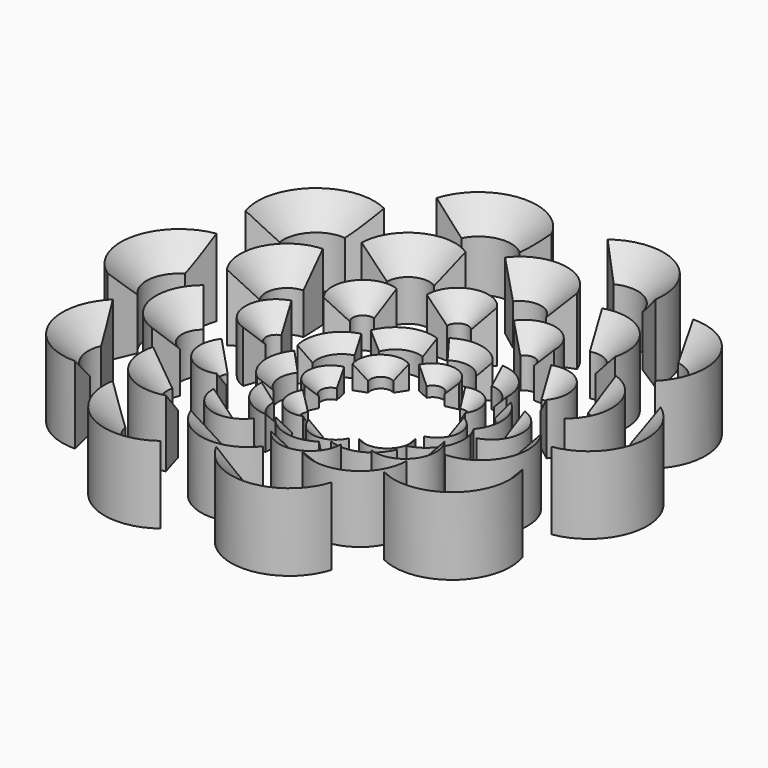
from build123d import *

# Parameters (mm, degrees)
F2_DEPTH       = 15
F3_DEPTH       = 13
F4_DEPTH       = 11
F5_DEPTH       = 9
F6_DEPTH       = 7
F7_T2_ANGLE    = 336.4519839088
F7_2_T2_ANGLE  = 359.64
F7_3_T2_ANGLE  = 336.4519839088
F7_4_T2_ANGLE  = 359.64
F7_5_T2_ANGLE  = 336.4519839088
F7_6_T2_ANGLE  = 336.4519839088
F7_7_T2_ANGLE  = 359.64
F7_8_T2_ANGLE  = 359.64
F7_9_T2_ANGLE  = 359.64
F7_10_T2_ANGLE = 359.64
F7_11_T2_ANGLE = 359.64
F7_12_T2_ANGLE = 359.64
F7_13_T2_ANGLE = 359.64
F7_14_T2_ANGLE = 336.4519839088
F7_15_T2_ANGLE = 336.4519839088
F7_16_T2_ANGLE = 359.64
F7_17_T2_ANGLE = 336.4519839088
F7_18_T2_ANGLE = 336.4519839088
F7_19_T2_ANGLE = 359.64
F7_20_T2_ANGLE = 359.64
F7_21_T2_ANGLE = 359.64
F7_22_T2_ANGLE = 359.64
F7_23_T2_ANGLE = 336.4519839088
F7_24_T2_ANGLE = 359.64
F7_25_T2_ANGLE = 359.64
F7_26_T2_ANGLE = 336.4519839088
F7_27_T2_ANGLE = 359.64
F7_28_T2_ANGLE = 359.64
F7_29_T2_ANGLE = 359.64
F7_30_T2_ANGLE = 359.64
F7_31_T2_ANGLE = 359.64
F7_32_T2_ANGLE = 359.64
F7_33_T2_ANGLE = 359.64
F7_34_T2_ANGLE = 359.64
F7_35_T2_ANGLE = 359.64
F7_36_T2_ANGLE = 359.64
F7_37_T2_ANGLE = 359.64
F7_38_T2_ANGLE = 359.64
F7_39_T2_ANGLE = 359.64
F7_40_T2_ANGLE = 359.64
F7_41_T2_ANGLE = 359.64
F7_42_T2_ANGLE = 359.64
F7_43_T2_ANGLE = 359.64
F7_44_T2_ANGLE = 359.64
F7_45_T2_ANGLE = 359.64
F7_46_T2_ANGLE = 359.64
F7_47_T2_ANGLE = 359.64
F7_48_T2_ANGLE = 359.64


# Not quite as in the source:
# - a fillet or chamfer that OpenCascade refuses, or shapes differently, is made with other operations: its cross-section is extruded or revolved along the edge and cut away or added


with BuildPart() as f2:
    # F1 (on offset) → F2 (new body)
    with BuildSketch(Plane.XY.offset(30)):
        with BuildLine():
            ThreePointArc((17.7590144577, -41.0240965166), (13.3006914412, -44.3521341763), (7.933868463, -42.8859520918))
            Line((7.933868463, -42.8859520918), (1.9961113601, -43.2368292953))
            ThreePointArc((1.9961113601, -43.2368292953), (13.0634500325, -49.4237184718), (22.9515977997, -41.487213151))
            Line((22.9515977997, -41.487213151), (17.7590144577, -41.0240965166))
        make_face()
    extrude(amount=F2_DEPTH)

    # F7#6: chamfer of 5 on 1 edges, made by hand

    # F7_6_s1 → F7_6_t2 (revolve, cut)
    with BuildSketch(Plane(origin=(12.8099025435, -0.2333815755, 0), x_dir=(0, 0, 1), z_dir=(-0.9998340782, 0.0182158179, 0))):
        Polygon((40, -31.5493184866), (45, -26.5493184866), (45, -31.5493184866), align=None)
    revolve(axis=Axis((12.1196571692, -38.1197312438, 45), (0, 0, -1)), revolution_arc=F7_6_T2_ANGLE, mode=Mode.SUBTRACT)


with BuildPart() as f2b:
    # F1 (on offset) → F2, piece 2 (new body)
    with BuildSketch(Plane.XY.offset(30)):
        with BuildLine():
            ThreePointArc((-9.7460144214, -43.6276780543), (-15.3090449637, -43.6995805599), (-18.7890957524, -39.3588749384))
            Line((-18.7890957524, -39.3588749384), (-23.7990826027, -36.1526145022))
            ThreePointArc((-23.7990826027, -36.1526145022), (-18.4819797497, -47.663131442), (-5.8173393808, -47.0544711917))
            Line((-5.8173393808, -47.0544711917), (-9.7460144214, -43.6276780543))
        make_face()
    extrude(amount=F2_DEPTH)

    # F7#5: chamfer of 5 on 1 edges, made by hand

    # F7_5_s1 → F7_5_t2 (revolve, cut)
    with BuildSketch(Plane(origin=(10.2262506057, -7.7182814591, 0), x_dir=(0, 0, 1), z_dir=(-0.7981757717, 0.6024246322, 0))):
        Polygon((40, -31.5493184866), (45, -26.5493184866), (45, -31.5493184866), align=None)
    revolve(axis=Axis((-12.6012072306, -37.9632661442, 45), (0, 0, -1)), revolution_arc=F7_5_T2_ANGLE, mode=Mode.SUBTRACT)


with BuildPart() as f2c:
    # F1 (on offset) → F2, piece 3 (new body)
    with BuildSketch(Plane.XY.offset(30)):
        with BuildLine():
            ThreePointArc((-33.5283970464, -29.5669694255), (-38.0712465277, -26.3552724637), (-38.3352640082, -20.7980453175))
            Line((-38.3352640082, -20.7980453175), (-40.5038359123, -15.2593297514))
            ThreePointArc((-40.5038359123, -15.2593297514), (-42.9679214469, -27.6968482117), (-32.364250642, -34.6485205598))
            Line((-32.364250642, -34.6485205598), (-33.5283970464, -29.5669694255))
        make_face()
    extrude(amount=F2_DEPTH)

    # F7#3: chamfer of 5 on 1 edges, made by hand

    # F7_3_s1 → F7_3_t2 (revolve, cut)
    with BuildSketch(Plane(origin=(3.7365185141, -12.2550601601, 0), x_dir=(0, 0, 1), z_dir=(-0.2916414494, 0.9565277126, 0))):
        Polygon((40, -31.5493184866), (45, -26.5493184866), (45, -31.5493184866), align=None)
    revolve(axis=Axis((-32.5088387676, -23.3061237014, 45), (0, 0, -1)), revolution_arc=F7_3_T2_ANGLE, mode=Mode.SUBTRACT)


with BuildPart() as f2d:
    # F1 (on offset) → F2, piece 4 (new body)
    with BuildSketch(Plane.XY.offset(30)):
        with BuildLine():
            ThreePointArc((-44.504071588, -4.2126834205), (-46.2915259123, 1.0558539309), (-43.2386643806, 5.7069307151))
            Line((-43.2386643806, 5.7069307151), (-41.7375005782, 11.4625003189))
            ThreePointArc((-41.7375005782, 11.4625003189), (-51.0415775773, 2.8486896542), (-46.5491181784, -9.0080127339))
            Line((-46.5491181784, -9.0080127339), (-44.504071588, -4.2126834205))
        make_face()
    extrude(amount=F2_DEPTH)

    # F7: chamfer of 5 on 1 edges, made by hand

    # F7_s1 → F7_t2 (revolve, cut)
    with BuildSketch(Plane(origin=(-4.1804366504, -12.1108224141, 0), x_dir=(0, 0, 1), z_dir=(0.3262899941, 0.945269718, 0))):
        Polygon((40, -31.5493184866), (45, -26.5493184866), (45, -31.5493184866), align=None)
    revolve(axis=Axis((-39.9991988301, 0.2531658493, 45), (0, 0, -1)), revolution_arc=F7_T2_ANGLE, mode=Mode.SUBTRACT)


with BuildPart() as f2e:
    # F1 (on offset) → F2, piece 5 (new body)
    with BuildSketch(Plane.XY.offset(30)):
        with BuildLine():
            ThreePointArc((-38.4807034207, 22.7507044673), (-36.8300157894, 28.063680011), (-31.6263645878, 30.032053186))
            Line((-31.6263645878, 30.032053186), (-27.0288586286, 33.8060448634))
            ThreePointArc((-27.0288586286, 33.8060448634), (-39.6190859126, 32.3061248957), (-42.9538047169, 20.0732497852))
            Line((-42.9538047169, 20.0732497852), (-38.4807034207, 22.7507044673))
        make_face()
    extrude(amount=F2_DEPTH)

    # F7#14: chamfer of 5 on 1 edges, made by hand

    # F7_14_s1 → F7_14_t2 (revolve, cut)
    with BuildSketch(Plane(origin=(-10.5006071022, -7.3406621376, 0), x_dir=(0, 0, 1), z_dir=(0.81958975, 0.5729508196, 0))):
        Polygon((40, -31.5493184866), (45, -26.5493184866), (45, -31.5493184866), align=None)
    revolve(axis=Axis((-32.2112244624, 23.7157546503, 45), (0, 0, -1)), revolution_arc=F7_14_T2_ANGLE, mode=Mode.SUBTRACT)


with BuildPart() as f2f:
    # F1 (on offset) → F2, piece 6 (new body)
    with BuildSketch(Plane.XY.offset(30)):
        with BuildLine():
            ThreePointArc((-17.7590144577, 41.0240965166), (-13.3006914412, 44.3521341763), (-7.933868463, 42.8859520918))
            Line((-7.933868463, 42.8859520918), (-1.9961113601, 43.2368292953))
            ThreePointArc((-1.9961113601, 43.2368292953), (-13.0634500325, 49.4237184718), (-22.9515977997, 41.487213151))
            Line((-22.9515977997, 41.487213151), (-17.7590144577, 41.0240965166))
        make_face()
    extrude(amount=F2_DEPTH)

    # F7#15: chamfer of 5 on 1 edges, made by hand

    # F7_15_s1 → F7_15_t2 (revolve, cut)
    with BuildSketch(Plane(origin=(-12.8099025435, 0.2333815755, 0), x_dir=(0, 0, 1), z_dir=(0.9998340782, -0.0182158179, 0))):
        Polygon((40, -31.5493184866), (45, -26.5493184866), (45, -31.5493184866), align=None)
    revolve(axis=Axis((-12.1196571692, 38.1197312438, 45), (0, 0, -1)), revolution_arc=F7_15_T2_ANGLE, mode=Mode.SUBTRACT)


with BuildPart() as f2g:
    # F1 (on offset) → F2, piece 7 (new body)
    with BuildSketch(Plane.XY.offset(30)):
        with BuildLine():
            ThreePointArc((9.7460144214, 43.6276780543), (15.3090449637, 43.6995805599), (18.7890957524, 39.3588749384))
            Line((18.7890957524, 39.3588749384), (23.7990826027, 36.1526145022))
            ThreePointArc((23.7990826027, 36.1526145022), (18.4819797497, 47.663131442), (5.8173393808, 47.0544711917))
            Line((5.8173393808, 47.0544711917), (9.7460144214, 43.6276780543))
        make_face()
    extrude(amount=F2_DEPTH)

    # F7#17: chamfer of 5 on 1 edges, made by hand

    # F7_17_s1 → F7_17_t2 (revolve, cut)
    with BuildSketch(Plane(origin=(-10.2262506057, 7.7182814591, 0), x_dir=(0, 0, 1), z_dir=(0.7981757717, -0.6024246322, 0))):
        Polygon((40, -31.5493184866), (45, -26.5493184866), (45, -31.5493184866), align=None)
    revolve(axis=Axis((12.6012072306, 37.9632661442, 45), (0, 0, -1)), revolution_arc=F7_17_T2_ANGLE, mode=Mode.SUBTRACT)


with BuildPart() as f2h:
    # F1 (on offset) → F2, piece 8 (new body)
    with BuildSketch(Plane.XY.offset(30)):
        with BuildLine():
            ThreePointArc((33.5283970464, 29.5669694255), (38.0712465277, 26.3552724637), (38.3352640082, 20.7980453175))
            Line((38.3352640082, 20.7980453175), (40.5038359123, 15.2593297514))
            ThreePointArc((40.5038359123, 15.2593297514), (42.9679214469, 27.6968482117), (32.364250642, 34.6485205598))
            Line((32.364250642, 34.6485205598), (33.5283970464, 29.5669694255))
        make_face()
    extrude(amount=F2_DEPTH)

    # F7#18: chamfer of 5 on 1 edges, made by hand

    # F7_18_s1 → F7_18_t2 (revolve, cut)
    with BuildSketch(Plane(origin=(-3.7365185141, 12.2550601601, 0), x_dir=(0, 0, 1), z_dir=(0.2916414494, -0.9565277126, 0))):
        Polygon((40, -31.5493184866), (45, -26.5493184866), (45, -31.5493184866), align=None)
    revolve(axis=Axis((32.5088387676, 23.3061237014, 45), (0, 0, -1)), revolution_arc=F7_18_T2_ANGLE, mode=Mode.SUBTRACT)


with BuildPart() as f2i:
    # F1 (on offset) → F2, piece 9 (new body)
    with BuildSketch(Plane.XY.offset(30)):
        with BuildLine():
            ThreePointArc((44.504071588, 4.2126834205), (46.2915259123, -1.0558539309), (43.2386643806, -5.7069307151))
            Line((43.2386643806, -5.7069307151), (41.7375005782, -11.4625003189))
            ThreePointArc((41.7375005782, -11.4625003189), (51.0415775773, -2.8486896542), (46.5491181784, 9.0080127339))
            Line((46.5491181784, 9.0080127339), (44.504071588, 4.2126834205))
        make_face()
    extrude(amount=F2_DEPTH)

    # F7#23: chamfer of 5 on 1 edges, made by hand

    # F7_23_s1 → F7_23_t2 (revolve, cut)
    with BuildSketch(Plane(origin=(4.1804366504, 12.1108224141, 0), x_dir=(0, 0, 1), z_dir=(-0.3262899941, -0.945269718, 0))):
        Polygon((40, -31.5493184866), (45, -26.5493184866), (45, -31.5493184866), align=None)
    revolve(axis=Axis((39.9991988301, -0.2531658493, 45), (0, 0, -1)), revolution_arc=F7_23_T2_ANGLE, mode=Mode.SUBTRACT)


with BuildPart() as f2j:
    # F1 (on offset) → F2, piece 10 (new body)
    with BuildSketch(Plane.XY.offset(30)):
        with BuildLine():
            ThreePointArc((38.4807034207, -22.7507044673), (36.8300157894, -28.063680011), (31.6263645878, -30.032053186))
            Line((31.6263645878, -30.032053186), (27.0288586286, -33.8060448634))
            ThreePointArc((27.0288586286, -33.8060448634), (39.6190859126, -32.3061248957), (42.9538047169, -20.0732497852))
            Line((42.9538047169, -20.0732497852), (38.4807034207, -22.7507044673))
        make_face()
    extrude(amount=F2_DEPTH)

    # F7#26: chamfer of 5 on 1 edges, made by hand

    # F7_26_s1 → F7_26_t2 (revolve, cut)
    with BuildSketch(Plane(origin=(10.5006071022, 7.3406621376, 0), x_dir=(0, 0, 1), z_dir=(-0.81958975, -0.5729508196, 0))):
        Polygon((40, -31.5493184866), (45, -26.5493184866), (45, -31.5493184866), align=None)
    revolve(axis=Axis((32.2112244624, -23.7157546503, 45), (0, 0, -1)), revolution_arc=F7_26_T2_ANGLE, mode=Mode.SUBTRACT)


with BuildPart() as f3:
    # F1 (on offset) → F3 (new body)
    with BuildSketch(Plane.XY.offset(30)):
        with BuildLine():
            Line((-6.1605418312, -31.6157678777), (-10.8426337183, -33.3701952944))
            ThreePointArc((-10.8426337183, -33.3701952944), (-3.5878071118, -39.2281581741), (5.0480977361, -35.7111444343))
            Line((5.0480977361, -35.7111444343), (1.0708378352, -32.6810613199))
            ThreePointArc((1.0708378352, -32.6810613199), (-2.8590949623, -34.2815453327), (-6.1605418312, -31.6157678777))
        make_face()
    extrude(amount=F3_DEPTH)

    # F7#7: chamfer of 5 on 1 edges, made by hand

    # F7_7_s1 → F7_7_t2 (revolve, cut)
    with BuildSketch(Plane(origin=(2.2372338796, -0.3367633156, 0), x_dir=(0, 0, 1), z_dir=(-0.9888598236, 0.1488497541, 0))):
        Polygon((38, -25.9742910378), (43, -20.9742910378), (43, -25.9742910378), align=None)
    revolve(axis=Axis((-2.2505512341, -30.1506546616, 43), (0, 0, -1)), revolution_arc=F7_7_T2_ANGLE, mode=Mode.SUBTRACT)


with BuildPart() as f3b:
    # F1 (on offset) → F3, piece 2 (new body)
    with BuildSketch(Plane.XY.offset(30)):
        with BuildLine():
            Line((-23.5672651344, -21.9566178688), (-28.3863836021, -20.6239149032))
            ThreePointArc((-28.3863836021, -20.6239149032), (-25.9603297754, -29.6273865125), (-16.9064871832, -31.8581201373))
            Line((-16.9064871832, -31.8581201373), (-18.3431198662, -27.0689566891))
            ThreePointArc((-18.3431198662, -27.0689566891), (-22.4632431853, -26.0538189138), (-23.5672651344, -21.9566178688))
        make_face()
    extrude(amount=F3_DEPTH)

    # F7#4: chamfer of 5 on 1 edges, made by hand

    # F7_4_s1 → F7_4_t2 (revolve, cut)
    with BuildSketch(Plane(origin=(1.6120157185, -1.5874603257, 0), x_dir=(0, 0, 1), z_dir=(-0.7125127121, 0.7016592016, 0))):
        Polygon((38, -25.9742910378), (43, -20.9742910378), (43, -25.9742910378), align=None)
    revolve(axis=Axis((-19.5428443521, -23.0695511878, 43), (0, 0, -1)), revolution_arc=F7_4_T2_ANGLE, mode=Mode.SUBTRACT)


with BuildPart() as f3c:
    # F1 (on offset) → F3, piece 3 (new body)
    with BuildSketch(Plane.XY.offset(30)):
        with BuildLine():
            Line((-31.9720941781, -3.910786112), (-35.0874997675, 0))
            ThreePointArc((-35.0874997675, 0), (-38.4168888238, -8.7099602009), (-32.4033686289, -15.8363767656))
            Line((-32.4033686289, -15.8363767656), (-30.7506292384, -11.1174306431))
            ThreePointArc((-30.7506292384, -11.1174306431), (-33.4871960092, -7.8744192066), (-31.9720941781, -3.910786112))
        make_face()
    extrude(amount=F3_DEPTH)

    # F7#2: chamfer of 5 on 1 edges, made by hand

    # F7_2_s1 → F7_2_t2 (revolve, cut)
    with BuildSketch(Plane(origin=(0.3710623434, -2.2318014472, 0), x_dir=(0, 0, 1), z_dir=(-0.164009962, 0.9864586826, 0))):
        Polygon((38, -25.9742910378), (43, -20.9742910378), (43, -25.9742910378), align=None)
    revolve(axis=Axis((-29.3704351645, -7.1766632655, 43), (0, 0, -1)), revolution_arc=F7_2_T2_ANGLE, mode=Mode.SUBTRACT)


with BuildPart() as f3d:
    # F1 (on offset) → F3, piece 4 (new body)
    with BuildSketch(Plane.XY.offset(30)):
        with BuildLine():
            Line((-28.1646699373, 15.6288330169), (-28.3863836021, 20.6239149032))
            ThreePointArc((-28.3863836021, 20.6239149032), (-36.1995020836, 15.5343748668), (-35.5232646083, 6.2343242719))
            Line((-35.5232646083, 6.2343242719), (-31.412443417, 9.080576041))
            ThreePointArc((-31.412443417, 9.080576041), (-31.7201781454, 13.3127409958), (-28.1646699373, 15.6288330169))
        make_face()
    extrude(amount=F3_DEPTH)

    # F7#12: chamfer of 5 on 1 edges, made by hand

    # F7_12_s1 → F7_12_t2 (revolve, cut)
    with BuildSketch(Plane(origin=(-1.0116242349, -2.023670272, 0), x_dir=(0, 0, 1), z_dir=(0.4471390191, 0.8944644753, 0))):
        Polygon((38, -25.9742910378), (43, -20.9742910378), (43, -25.9742910378), align=None)
    revolve(axis=Axis((-27.9795180084, 11.4574660984, 43), (0, 0, -1)), revolution_arc=F7_12_T2_ANGLE, mode=Mode.SUBTRACT)


with BuildPart() as f3e:
    # F1 (on offset) → F3, piece 5 (new body)
    with BuildSketch(Plane.XY.offset(30)):
        with BuildLine():
            Line((-13.5992990624, 29.1987691378), (-10.8426337183, 33.3701952944))
            ThreePointArc((-10.8426337183, 33.3701952944), (-20.1551359233, 33.8451067293), (-25.0744808987, 25.9237253345))
            Line((-25.0744808987, 25.9237253345), (-20.07577188, 25.8101113149))
            ThreePointArc((-20.07577188, 25.8101113149), (-17.8371303593, 29.4148866213), (-13.5992990624, 29.1987691378))
        make_face()
    extrude(amount=F3_DEPTH)

    # F7#13: chamfer of 5 on 1 edges, made by hand

    # F7_13_s1 → F7_13_t2 (revolve, cut)
    with BuildSketch(Plane(origin=(-2.0079047394, -1.0425658349, 0), x_dir=(0, 0, 1), z_dir=(0.8874960926, 0.4608152402, 0))):
        Polygon((38, -25.9742910378), (43, -20.9742910378), (43, -25.9742910378), align=None)
    revolve(axis=Axis((-15.901375962, 25.7152328377, 43), (0, 0, -1)), revolution_arc=F7_13_T2_ANGLE, mode=Mode.SUBTRACT)


with BuildPart() as f3f:
    # F1 (on offset) → F3, piece 6 (new body)
    with BuildSketch(Plane.XY.offset(30)):
        with BuildLine():
            Line((6.1605418312, 31.6157678777), (10.8426337183, 33.3701952944))
            ThreePointArc((10.8426337183, 33.3701952944), (3.5878071118, 39.2281581741), (-5.0480977361, 35.7111444343))
            Line((-5.0480977361, 35.7111444343), (-1.0708378352, 32.6810613199))
            ThreePointArc((-1.0708378352, 32.6810613199), (2.8590949623, 34.2815453327), (6.1605418312, 31.6157678777))
        make_face()
    extrude(amount=F3_DEPTH)

    # F7#16: chamfer of 5 on 1 edges, made by hand

    # F7_16_s1 → F7_16_t2 (revolve, cut)
    with BuildSketch(Plane(origin=(-2.2372338796, 0.3367633156, 0), x_dir=(0, 0, 1), z_dir=(0.9888598236, -0.1488497541, 0))):
        Polygon((38, -25.9742910378), (43, -20.9742910378), (43, -25.9742910378), align=None)
    revolve(axis=Axis((2.2505512341, 30.1506546616, 43), (0, 0, -1)), revolution_arc=F7_16_T2_ANGLE, mode=Mode.SUBTRACT)


with BuildPart() as f3g:
    # F1 (on offset) → F3, piece 7 (new body)
    with BuildSketch(Plane.XY.offset(30)):
        with BuildLine():
            Line((23.5672651344, 21.9566178688), (28.3863836021, 20.6239149032))
            ThreePointArc((28.3863836021, 20.6239149032), (25.9603297754, 29.6273865125), (16.9064871832, 31.8581201373))
            Line((16.9064871832, 31.8581201373), (18.3431198662, 27.0689566891))
            ThreePointArc((18.3431198662, 27.0689566891), (22.4632431853, 26.0538189138), (23.5672651344, 21.9566178688))
        make_face()
    extrude(amount=F3_DEPTH)

    # F7#19: chamfer of 5 on 1 edges, made by hand

    # F7_19_s1 → F7_19_t2 (revolve, cut)
    with BuildSketch(Plane(origin=(-1.6120157185, 1.5874603257, 0), x_dir=(0, 0, 1), z_dir=(0.7125127121, -0.7016592016, 0))):
        Polygon((38, -25.9742910378), (43, -20.9742910378), (43, -25.9742910378), align=None)
    revolve(axis=Axis((19.5428443521, 23.0695511878, 43), (0, 0, -1)), revolution_arc=F7_19_T2_ANGLE, mode=Mode.SUBTRACT)


with BuildPart() as f3h:
    # F1 (on offset) → F3, piece 8 (new body)
    with BuildSketch(Plane.XY.offset(30)):
        with BuildLine():
            Line((31.9720941781, 3.910786112), (35.0874997675, 0))
            ThreePointArc((35.0874997675, 0), (38.4168888238, 8.7099602009), (32.4033686289, 15.8363767656))
            Line((32.4033686289, 15.8363767656), (30.7506292384, 11.1174306431))
            ThreePointArc((30.7506292384, 11.1174306431), (33.4871960092, 7.8744192066), (31.9720941781, 3.910786112))
        make_face()
    extrude(amount=F3_DEPTH)

    # F7#22: chamfer of 5 on 1 edges, made by hand

    # F7_22_s1 → F7_22_t2 (revolve, cut)
    with BuildSketch(Plane(origin=(-0.3710623434, 2.2318014472, 0), x_dir=(0, 0, 1), z_dir=(0.164009962, -0.9864586826, 0))):
        Polygon((38, -25.9742910378), (43, -20.9742910378), (43, -25.9742910378), align=None)
    revolve(axis=Axis((29.3704351645, 7.1766632655, 43), (0, 0, -1)), revolution_arc=F7_22_T2_ANGLE, mode=Mode.SUBTRACT)


with BuildPart() as f3i:
    # F1 (on offset) → F3, piece 9 (new body)
    with BuildSketch(Plane.XY.offset(30)):
        with BuildLine():
            Line((28.1646699373, -15.6288330169), (28.3863836021, -20.6239149032))
            ThreePointArc((28.3863836021, -20.6239149032), (36.1995020836, -15.5343748668), (35.5232646083, -6.2343242719))
            Line((35.5232646083, -6.2343242719), (31.412443417, -9.080576041))
            ThreePointArc((31.412443417, -9.080576041), (31.7201781454, -13.3127409958), (28.1646699373, -15.6288330169))
        make_face()
    extrude(amount=F3_DEPTH)

    # F7#25: chamfer of 5 on 1 edges, made by hand

    # F7_25_s1 → F7_25_t2 (revolve, cut)
    with BuildSketch(Plane(origin=(1.0116242349, 2.023670272, 0), x_dir=(0, 0, 1), z_dir=(-0.4471390191, -0.8944644753, 0))):
        Polygon((38, -25.9742910378), (43, -20.9742910378), (43, -25.9742910378), align=None)
    revolve(axis=Axis((27.9795180084, -11.4574660984, 43), (0, 0, -1)), revolution_arc=F7_25_T2_ANGLE, mode=Mode.SUBTRACT)


with BuildPart() as f3j:
    # F1 (on offset) → F3, piece 10 (new body)
    with BuildSketch(Plane.XY.offset(30)):
        with BuildLine():
            Line((13.5992990624, -29.1987691378), (10.8426337183, -33.3701952944))
            ThreePointArc((10.8426337183, -33.3701952944), (20.1551359233, -33.8451067293), (25.0744808987, -25.9237253345))
            Line((25.0744808987, -25.9237253345), (20.07577188, -25.8101113149))
            ThreePointArc((20.07577188, -25.8101113149), (17.8371303593, -29.4148866213), (13.5992990624, -29.1987691378))
        make_face()
    extrude(amount=F3_DEPTH)

    # F7#29: chamfer of 5 on 1 edges, made by hand

    # F7_29_s1 → F7_29_t2 (revolve, cut)
    with BuildSketch(Plane(origin=(2.0079047394, 1.0425658349, 0), x_dir=(0, 0, 1), z_dir=(-0.8874960926, -0.4608152402, 0))):
        Polygon((38, -25.9742910378), (43, -20.9742910378), (43, -25.9742910378), align=None)
    revolve(axis=Axis((15.901375962, -25.7152328377, 43), (0, 0, -1)), revolution_arc=F7_29_T2_ANGLE, mode=Mode.SUBTRACT)


with BuildPart() as f4:
    # F1 (on offset) → F4 (new body)
    with BuildSketch(Plane.XY.offset(30)):
        with BuildLine():
            Line((16.4369760922, -18.1697884033), (15.0690451836, -21.9286240894))
            ThreePointArc((15.0690451836, -21.9286240894), (21.9202890216, -19.9036330194), (21.9774614573, -12.7596241817))
            Line((21.9774614573, -12.7596241817), (18.6972737041, -15.0528288908))
            ThreePointArc((18.6972737041, -15.0528288908), (18.7473416536, -17.4671558607), (16.4369760922, -18.1697884033))
        make_face()
    extrude(amount=F4_DEPTH)

    # F7#28: chamfer of 5 on 1 edges, made by hand

    # F7_28_s1 → F7_28_t2 (revolve, cut)
    with BuildSketch(Plane(origin=(-1.8048632112, -2.4725317677, 0), x_dir=(0, 0, 1), z_dir=(-0.5895933936, -0.8077002106, 0))):
        Polygon((36, -21.4407613721), (41, -16.4407613721), (41, -21.4407613721), align=None)
    revolve(axis=Axis((17.1282446856, -16.2930498142, 41), (0, 0, -1)), revolution_arc=F7_28_T2_ANGLE, mode=Mode.SUBTRACT)


with BuildPart() as f4b:
    # F1 (on offset) → F4, piece 2 (new body)
    with BuildSketch(Plane.XY.offset(30)):
        with BuildLine():
            Line((2.617859334, -24.3610797418), (-0.6982082003, -26.5979920766))
            ThreePointArc((-0.6982082003, -26.5979920766), (6.0348243842, -28.9867999754), (10.2802208934, -23.2407805322))
            Line((10.2802208934, -23.2407805322), (6.2785813478, -23.1679761274))
            ThreePointArc((6.2785813478, -23.1679761274), (4.8999813827, -25.1506368783), (2.617859334, -24.3610797418))
        make_face()
    extrude(amount=F4_DEPTH)

    # F7#30: chamfer of 5 on 1 edges, made by hand

    # F7_30_s1 → F7_30_t2 (revolve, cut)
    with BuildSketch(Plane(origin=(-2.9134827193, -0.9394482413, 0), x_dir=(0, 0, 1), z_dir=(-0.9517453473, -0.3068888951, 0))):
        Polygon((36, -21.4407613721), (41, -16.4407613721), (41, -21.4407613721), align=None)
    revolve(axis=Axis((4.2802266388, -23.2490838137, 41), (0, 0, -1)), revolution_arc=F7_30_T2_ANGLE, mode=Mode.SUBTRACT)


with BuildPart() as f4c:
    # F1 (on offset) → F4, piece 3 (new body)
    with BuildSketch(Plane.XY.offset(30)):
        with BuildLine():
            Line((-12.2011907121, -21.2472666215), (-16.1987697829, -21.1078311231))
            ThreePointArc((-16.1987697829, -21.1078311231), (-12.1557380518, -26.9979945659), (-5.3437146399, -24.8447486446))
            Line((-5.3437146399, -24.8447486446), (-8.5383156822, -22.433743934))
            ThreePointArc((-8.5383156822, -22.433743934), (-10.8190052321, -23.2274294472), (-12.2011907121, -21.2472666215))
        make_face()
    extrude(amount=F4_DEPTH)

    # F7#8: chamfer of 5 on 1 edges, made by hand

    # F7_8_s1 → F7_8_t2 (revolve, cut)
    with BuildSketch(Plane(origin=(-2.9092508542, 0.9524725827, 0), x_dir=(0, 0, 1), z_dir=(-0.9503629269, 0.3111435475, 0))):
        Polygon((36, -21.4407613721), (41, -16.4407613721), (41, -21.4407613721), align=None)
    revolve(axis=Axis((-10.2026925045, -21.3247580037, 41), (0, 0, -1)), revolution_arc=F7_8_T2_ANGLE, mode=Mode.SUBTRACT)


with BuildPart() as f4d:
    # F1 (on offset) → F4, piece 4 (new body)
    with BuildSketch(Plane.XY.offset(30)):
        with BuildLine():
            Line((-22.3598006093, -10.0177198199), (-25.5119518843, -7.5551961093))
            ThreePointArc((-25.5119518843, -7.5551961093), (-25.7032217104, -14.6968728602), (-18.926532807, -16.9588672166))
            Line((-18.926532807, -16.9588672166), (-20.0938663283, -13.1305840526))
            ThreePointArc((-20.0938663283, -13.1305840526), (-22.4054995727, -12.4321334385), (-22.3598006093, -10.0177198199))
        make_face()
    extrude(amount=F4_DEPTH)

    # F7#9: chamfer of 5 on 1 edges, made by hand

    # F7_9_s1 → F7_9_t2 (revolve, cut)
    with BuildSketch(Plane(origin=(-1.7937840447, 2.4805812534, 0), x_dir=(0, 0, 1), z_dir=(-0.5859741701, 0.8103297304, 0))):
        Polygon((36, -21.4407613721), (41, -16.4407613721), (41, -21.4407613721), align=None)
    revolve(axis=Axis((-20.7885298878, -11.2550994381, 41), (0, 0, -1)), revolution_arc=F7_9_T2_ANGLE, mode=Mode.SUBTRACT)


with BuildPart() as f4e:
    # F1 (on offset) → F4, piece 5 (new body)
    with BuildSketch(Plane.XY.offset(30)):
        with BuildLine():
            Line((-23.9777266555, 5.0382554632), (-25.0804354853, 8.8832670265))
            ThreePointArc((-25.0804354853, 8.8832670265), (-29.4329482959, 3.2179547496), (-25.280058731, -2.5952749226))
            Line((-25.280058731, -2.5952749226), (-23.9742430024, 1.1880126447))
            ThreePointArc((-23.9742430024, 1.1880126447), (-25.4338546115, 3.111814991), (-23.9777266555, 5.0382554632))
        make_face()
    extrude(amount=F4_DEPTH)

    # F7#10: chamfer of 5 on 1 edges, made by hand

    # F7_10_s1 → F7_10_t2 (revolve, cut)
    with BuildSketch(Plane(origin=(0.0068473015, 3.0611921972, 0), x_dir=(0, 0, 1), z_dir=(0.0022368032, 0.9999974984, 0))):
        Polygon((36, -21.4407613721), (41, -16.4407613721), (41, -21.4407613721), align=None)
    revolve(axis=Axis((-23.4338554301, 3.1136245661, 41), (0, 0, -1)), revolution_arc=F7_10_T2_ANGLE, mode=Mode.SUBTRACT)


with BuildPart() as f4f:
    # F1 (on offset) → F4, piece 6 (new body)
    with BuildSketch(Plane.XY.offset(30)):
        with BuildLine():
            Line((-16.4369760922, 18.1697884033), (-15.0690451836, 21.9286240894))
            ThreePointArc((-15.0690451836, 21.9286240894), (-21.9202890216, 19.9036330194), (-21.9774614573, 12.7596241817))
            Line((-21.9774614573, 12.7596241817), (-18.6972737041, 15.0528288908))
            ThreePointArc((-18.6972737041, 15.0528288908), (-18.7473416536, 17.4671558607), (-16.4369760922, 18.1697884033))
        make_face()
    extrude(amount=F4_DEPTH)

    # F7#11: chamfer of 5 on 1 edges, made by hand

    # F7_11_s1 → F7_11_t2 (revolve, cut)
    with BuildSketch(Plane(origin=(1.8048632112, 2.4725317677, 0), x_dir=(0, 0, 1), z_dir=(0.5895933936, 0.8077002106, 0))):
        Polygon((36, -21.4407613721), (41, -16.4407613721), (41, -21.4407613721), align=None)
    revolve(axis=Axis((-17.1282446856, 16.2930498142, 41), (0, 0, -1)), revolution_arc=F7_11_T2_ANGLE, mode=Mode.SUBTRACT)


with BuildPart() as f4g:
    # F1 (on offset) → F4, piece 7 (new body)
    with BuildSketch(Plane.XY.offset(30)):
        with BuildLine():
            Line((-2.617859334, 24.3610797418), (0.6982082003, 26.5979920766))
            ThreePointArc((0.6982082003, 26.5979920766), (-6.0348243842, 28.9867999754), (-10.2802208934, 23.2407805322))
            Line((-10.2802208934, 23.2407805322), (-6.2785813478, 23.1679761274))
            ThreePointArc((-6.2785813478, 23.1679761274), (-4.8999813827, 25.1506368783), (-2.617859334, 24.3610797418))
        make_face()
    extrude(amount=F4_DEPTH)

    # F7#20: chamfer of 5 on 1 edges, made by hand

    # F7_20_s1 → F7_20_t2 (revolve, cut)
    with BuildSketch(Plane(origin=(2.9134827193, 0.9394482413, 0), x_dir=(0, 0, 1), z_dir=(0.9517453473, 0.3068888951, 0))):
        Polygon((36, -21.4407613721), (41, -16.4407613721), (41, -21.4407613721), align=None)
    revolve(axis=Axis((-4.2802266388, 23.2490838137, 41), (0, 0, -1)), revolution_arc=F7_20_T2_ANGLE, mode=Mode.SUBTRACT)


with BuildPart() as f4h:
    # F1 (on offset) → F4, piece 8 (new body)
    with BuildSketch(Plane.XY.offset(30)):
        with BuildLine():
            Line((12.2011907121, 21.2472666215), (16.1987697829, 21.1078311231))
            ThreePointArc((16.1987697829, 21.1078311231), (12.1557380518, 26.9979945659), (5.3437146399, 24.8447486446))
            Line((5.3437146399, 24.8447486446), (8.5383156822, 22.433743934))
            ThreePointArc((8.5383156822, 22.433743934), (10.8190052321, 23.2274294472), (12.2011907121, 21.2472666215))
        make_face()
    extrude(amount=F4_DEPTH)

    # F7#21: chamfer of 5 on 1 edges, made by hand

    # F7_21_s1 → F7_21_t2 (revolve, cut)
    with BuildSketch(Plane(origin=(2.9092508542, -0.9524725827, 0), x_dir=(0, 0, 1), z_dir=(0.9503629269, -0.3111435475, 0))):
        Polygon((36, -21.4407613721), (41, -16.4407613721), (41, -21.4407613721), align=None)
    revolve(axis=Axis((10.2026925045, 21.3247580037, 41), (0, 0, -1)), revolution_arc=F7_21_T2_ANGLE, mode=Mode.SUBTRACT)


with BuildPart() as f4i:
    # F1 (on offset) → F4, piece 9 (new body)
    with BuildSketch(Plane.XY.offset(30)):
        with BuildLine():
            Line((22.3598006093, 10.0177198199), (25.5119518843, 7.5551961093))
            ThreePointArc((25.5119518843, 7.5551961093), (25.7032217104, 14.6968728602), (18.926532807, 16.9588672166))
            Line((18.926532807, 16.9588672166), (20.0938663283, 13.1305840526))
            ThreePointArc((20.0938663283, 13.1305840526), (22.4054995727, 12.4321334385), (22.3598006093, 10.0177198199))
        make_face()
    extrude(amount=F4_DEPTH)

    # F7#24: chamfer of 5 on 1 edges, made by hand

    # F7_24_s1 → F7_24_t2 (revolve, cut)
    with BuildSketch(Plane(origin=(1.7937840447, -2.4805812534, 0), x_dir=(0, 0, 1), z_dir=(0.5859741701, -0.8103297304, 0))):
        Polygon((36, -21.4407613721), (41, -16.4407613721), (41, -21.4407613721), align=None)
    revolve(axis=Axis((20.7885298878, 11.2550994381, 41), (0, 0, -1)), revolution_arc=F7_24_T2_ANGLE, mode=Mode.SUBTRACT)


with BuildPart() as f4j:
    # F1 (on offset) → F4, piece 10 (new body)
    with BuildSketch(Plane.XY.offset(30)):
        with BuildLine():
            Line((23.9777266555, -5.0382554632), (25.0804354853, -8.8832670265))
            ThreePointArc((25.0804354853, -8.8832670265), (29.4329482959, -3.2179547496), (25.280058731, 2.5952749226))
            Line((25.280058731, 2.5952749226), (23.9742430024, -1.1880126447))
            ThreePointArc((23.9742430024, -1.1880126447), (25.4338546115, -3.111814991), (23.9777266555, -5.0382554632))
        make_face()
    extrude(amount=F4_DEPTH)

    # F7#27: chamfer of 5 on 1 edges, made by hand

    # F7_27_s1 → F7_27_t2 (revolve, cut)
    with BuildSketch(Plane(origin=(-0.0068473015, -3.0611921972, 0), x_dir=(0, 0, 1), z_dir=(-0.0022368032, -0.9999974984, 0))):
        Polygon((36, -21.4407613721), (41, -16.4407613721), (41, -21.4407613721), align=None)
    revolve(axis=Axis((23.4338554301, -3.1136245661, 41), (0, 0, -1)), revolution_arc=F7_27_T2_ANGLE, mode=Mode.SUBTRACT)


with BuildPart() as f5:
    # F1 (on offset) → F5 (new body)
    with BuildSketch(Plane.XY.offset(30)):
        with BuildLine():
            ThreePointArc((11.4574590961, -13.1497890945), (8.908938927, -15.8437013251), (5.2012266489, -15.9143258353))
            Line((5.2012266489, -15.9143258353), (4.2785849826, -18.2378430734))
            ThreePointArc((4.2785849826, -18.2378430734), (9.9193959352, -18.1303968962), (13.7966440614, -14.0319533072))
            Line((13.7966440614, -14.0319533072), (11.4574590961, -13.1497890945))
        make_face()
    extrude(amount=F5_DEPTH)

    # F7#33: chamfer of 5 on 1 edges, made by hand

    # F7_33_s1 → F7_33_t2 (revolve, cut)
    with BuildSketch(Plane(origin=(1.6366335731, 0.7170671044, 0), x_dir=(0, 0, 1), z_dir=(-0.9159434903, -0.401307267, 0))):
        Polygon((34, -8.4971056244), (39, -3.4971056244), (39, -8.4971056244), align=None)
    revolve(axis=Axis((6.9708672159, -11.457784891, 39), (0, 0, -1)), revolution_arc=F7_33_T2_ANGLE, mode=Mode.SUBTRACT)


with BuildPart() as f5b:
    # F1 (on offset) → F5, piece 2 (new body)
    with BuildSketch(Plane.XY.offset(30)):
        with BuildLine():
            ThreePointArc((1.5400270206, -17.3729283353), (-2.1052109868, -18.0543665407), (-5.1463252756, -15.9321643728))
            Line((-5.1463252756, -15.9321643728), (-7.2584872294, -17.2696141406))
            ThreePointArc((-7.2584872294, -17.2696141406), (-2.6318200283, -20.4982738461), (2.9139442962, -19.4615526003))
            Line((2.9139442962, -19.4615526003), (1.5400270206, -17.3729283353))
        make_face()
    extrude(amount=F5_DEPTH)

    # F7#32: chamfer of 5 on 1 edges, made by hand

    # F7_32_s1 → F7_32_t2 (revolve, cut)
    with BuildSketch(Plane(origin=(1.745545843, -0.3818696041, 0), x_dir=(0, 0, 1), z_dir=(-0.9768963427, 0.2137136765, 0))):
        Polygon((34, -8.4971056244), (39, -3.4971056244), (39, -8.4971056244), align=None)
    revolve(axis=Axis((-1.0951669397, -13.3669156399, 39), (0, 0, -1)), revolution_arc=F7_32_T2_ANGLE, mode=Mode.SUBTRACT)


with BuildPart() as f5c:
    # F1 (on offset) → F5, piece 3 (new body)
    with BuildSketch(Plane.XY.offset(30)):
        with BuildLine():
            ThreePointArc((-8.9656430332, -14.9601994362), (-12.3152418572, -13.3688773831), (-13.528155862, -9.8644576343))
            Line((-13.528155862, -9.8644576343), (-16.0230640266, -9.7049795786))
            ThreePointArc((-16.0230640266, -9.7049795786), (-14.1777701932, -15.0365068976), (-9.0817831489, -17.4575002738))
            Line((-9.0817831489, -17.4575002738), (-8.9656430332, -14.9601994362))
        make_face()
    extrude(amount=F5_DEPTH)

    # F7#31: chamfer of 5 on 1 edges, made by hand

    # F7_31_s1 → F7_31_t2 (revolve, cut)
    with BuildSketch(Plane(origin=(1.1877189299, -1.3349451031, 0), x_dir=(0, 0, 1), z_dir=(-0.6647079957, 0.7471032595, 0))):
        Polygon((34, -8.4971056244), (39, -3.4971056244), (39, -8.4971056244), align=None)
    revolve(axis=Axis((-8.7428845477, -10.1703389391, 39), (0, 0, -1)), revolution_arc=F7_31_T2_ANGLE, mode=Mode.SUBTRACT)


with BuildPart() as f5d:
    # F1 (on offset) → F5, piece 4 (new body)
    with BuildSketch(Plane.XY.offset(30)):
        with BuildLine():
            ThreePointArc((-16.0467421793, -6.8331828309), (-17.8212689178, -3.5769314565), (-16.7426907142, -0.02886336))
            Line((-16.7426907142, -0.02886336), (-18.6673749696, 1.5666273222))
            ThreePointArc((-18.6673749696, 1.5666273222), (-20.308294029, -3.8313053862), (-17.6085781095, -8.7852762014))
            Line((-17.6085781095, -8.7852762014), (-16.0467421793, -6.8331828309))
        make_face()
    extrude(amount=F5_DEPTH)

    # F7#40: chamfer of 5 on 1 edges, made by hand

    # F7_40_s1 → F7_40_t2 (revolve, cut)
    with BuildSketch(Plane(origin=(0.1762237546, -1.7781169458, 0), x_dir=(0, 0, 1), z_dir=(-0.098623787, 0.9951247905, 0))):
        Polygon((34, -8.4971056244), (39, -3.4971056244), (39, -8.4971056244), align=None)
    revolve(axis=Axis((-13.0511174182, -3.0890384407, 39), (0, 0, -1)), revolution_arc=F7_40_T2_ANGLE, mode=Mode.SUBTRACT)


with BuildPart() as f5e:
    # F1 (on offset) → F5, piece 5 (new body)
    with BuildSketch(Plane.XY.offset(30)):
        with BuildLine():
            Line((-13.5620867767, 9.8177557367), (-14.181383155, 12.2398358337))
            ThreePointArc((-14.181383155, 12.2398358337), (-18.6817397993, 8.8373245614), (-19.4094947259, 3.2426247794))
            Line((-19.4094947259, 3.2426247794), (-16.9985312216, 3.9038773644))
            ThreePointArc((-16.9985312216, 3.9038773644), (-16.5201769745, 7.581280711), (-13.5620867767, 9.8177557367))
        make_face()
    extrude(amount=F5_DEPTH)

    # F7#39: chamfer of 5 on 1 edges, made by hand

    # F7_39_s1 → F7_39_t2 (revolve, cut)
    with BuildSketch(Plane(origin=(-0.9025829053, -1.5421085512, 0), x_dir=(0, 0, 1), z_dir=(0.5051313563, 0.8630424745, 0))):
        Polygon((34, -8.4971056244), (39, -3.4971056244), (39, -8.4971056244), align=None)
    revolve(axis=Axis((-12.3742670261, 5.1721697495, 39), (0, 0, -1)), revolution_arc=F7_39_T2_ANGLE, mode=Mode.SUBTRACT)


with BuildPart() as f5f:
    # F1 (on offset) → F5, piece 6 (new body)
    with BuildSketch(Plane.XY.offset(30)):
        with BuildLine():
            ThreePointArc((-11.4574590961, 13.1497890945), (-8.908938927, 15.8437013251), (-5.2012266489, 15.9143258353))
            Line((-5.2012266489, 15.9143258353), (-4.2785849826, 18.2378430734))
            ThreePointArc((-4.2785849826, 18.2378430734), (-9.9193959352, 18.1303968962), (-13.7966440614, 14.0319533072))
            Line((-13.7966440614, 14.0319533072), (-11.4574590961, 13.1497890945))
        make_face()
    extrude(amount=F5_DEPTH)

    # F7#38: chamfer of 5 on 1 edges, made by hand

    # F7_38_s1 → F7_38_t2 (revolve, cut)
    with BuildSketch(Plane(origin=(-1.6366335731, -0.7170671044, 0), x_dir=(0, 0, 1), z_dir=(0.9159434903, 0.401307267, 0))):
        Polygon((34, -8.4971056244), (39, -3.4971056244), (39, -8.4971056244), align=None)
    revolve(axis=Axis((-6.9708672159, 11.457784891, 39), (0, 0, -1)), revolution_arc=F7_38_T2_ANGLE, mode=Mode.SUBTRACT)


with BuildPart() as f5g:
    # F1 (on offset) → F5, piece 7 (new body)
    with BuildSketch(Plane.XY.offset(30)):
        with BuildLine():
            ThreePointArc((-1.5400270206, 17.3729283353), (2.1052109868, 18.0543665407), (5.1463252756, 15.9321643728))
            Line((5.1463252756, 15.9321643728), (7.2584872294, 17.2696141406))
            ThreePointArc((7.2584872294, 17.2696141406), (2.6318200283, 20.4982738461), (-2.9139442962, 19.4615526003))
            Line((-2.9139442962, 19.4615526003), (-1.5400270206, 17.3729283353))
        make_face()
    extrude(amount=F5_DEPTH)

    # F7#37: chamfer of 5 on 1 edges, made by hand

    # F7_37_s1 → F7_37_t2 (revolve, cut)
    with BuildSketch(Plane(origin=(-1.745545843, 0.3818696041, 0), x_dir=(0, 0, 1), z_dir=(0.9768963427, -0.2137136765, 0))):
        Polygon((34, -8.4971056244), (39, -3.4971056244), (39, -8.4971056244), align=None)
    revolve(axis=Axis((1.0951669397, 13.3669156399, 39), (0, 0, -1)), revolution_arc=F7_37_T2_ANGLE, mode=Mode.SUBTRACT)


with BuildPart() as f5h:
    # F1 (on offset) → F5, piece 8 (new body)
    with BuildSketch(Plane.XY.offset(30)):
        with BuildLine():
            ThreePointArc((8.9656430332, 14.9601994362), (12.3152418572, 13.3688773831), (13.528155862, 9.8644576343))
            Line((13.528155862, 9.8644576343), (16.0230640266, 9.7049795786))
            ThreePointArc((16.0230640266, 9.7049795786), (14.1777701932, 15.0365068976), (9.0817831489, 17.4575002738))
            Line((9.0817831489, 17.4575002738), (8.9656430332, 14.9601994362))
        make_face()
    extrude(amount=F5_DEPTH)

    # F7#36: chamfer of 5 on 1 edges, made by hand

    # F7_36_s1 → F7_36_t2 (revolve, cut)
    with BuildSketch(Plane(origin=(-1.1877189299, 1.3349451031, 0), x_dir=(0, 0, 1), z_dir=(0.6647079957, -0.7471032595, 0))):
        Polygon((34, -8.4971056244), (39, -3.4971056244), (39, -8.4971056244), align=None)
    revolve(axis=Axis((8.7428845477, 10.1703389391, 39), (0, 0, -1)), revolution_arc=F7_36_T2_ANGLE, mode=Mode.SUBTRACT)


with BuildPart() as f5i:
    # F1 (on offset) → F5, piece 9 (new body)
    with BuildSketch(Plane.XY.offset(30)):
        with BuildLine():
            ThreePointArc((16.0467421793, 6.8331828309), (17.8212689178, 3.5769314565), (16.7426907142, 0.02886336))
            Line((16.7426907142, 0.02886336), (18.6673749696, -1.5666273222))
            ThreePointArc((18.6673749696, -1.5666273222), (20.308294029, 3.8313053862), (17.6085781095, 8.7852762014))
            Line((17.6085781095, 8.7852762014), (16.0467421793, 6.8331828309))
        make_face()
    extrude(amount=F5_DEPTH)

    # F7#35: chamfer of 5 on 1 edges, made by hand

    # F7_35_s1 → F7_35_t2 (revolve, cut)
    with BuildSketch(Plane(origin=(-0.1762237546, 1.7781169458, 0), x_dir=(0, 0, 1), z_dir=(0.098623787, -0.9951247905, 0))):
        Polygon((34, -8.4971056244), (39, -3.4971056244), (39, -8.4971056244), align=None)
    revolve(axis=Axis((13.0511174182, 3.0890384407, 39), (0, 0, -1)), revolution_arc=F7_35_T2_ANGLE, mode=Mode.SUBTRACT)


with BuildPart() as f5j:
    # F1 (on offset) → F5, piece 10 (new body)
    with BuildSketch(Plane.XY.offset(30)):
        with BuildLine():
            ThreePointArc((16.9985312216, -3.9038773644), (16.5201769745, -7.581280711), (13.5620867767, -9.8177557367))
            Line((13.5620867767, -9.8177557367), (14.181383155, -12.2398358337))
            ThreePointArc((14.181383155, -12.2398358337), (18.6817397993, -8.8373245614), (19.4094947259, -3.2426247794))
            Line((19.4094947259, -3.2426247794), (16.9985312216, -3.9038773644))
        make_face()
    extrude(amount=F5_DEPTH)

    # F7#34: chamfer of 5 on 1 edges, made by hand

    # F7_34_s1 → F7_34_t2 (revolve, cut)
    with BuildSketch(Plane(origin=(0.9025829053, 1.5421085512, 0), x_dir=(0, 0, 1), z_dir=(-0.5051313563, -0.8630424745, 0))):
        Polygon((34, -8.4971056244), (39, -3.4971056244), (39, -8.4971056244), align=None)
    revolve(axis=Axis((12.3742670261, -5.1721697495, 39), (0, 0, -1)), revolution_arc=F7_34_T2_ANGLE, mode=Mode.SUBTRACT)


with BuildPart() as f6:
    # F1 (on offset) → F6 (new body)
    with BuildSketch(Plane.XY.offset(30)):
        with BuildLine():
            Line((6.1107423525, -9.8856449278), (4.7406773223, -11.9767981535))
            ThreePointArc((4.7406773223, -11.9767981535), (10.0125562584, -11.7309179449), (11.4252081572, -6.6458831165))
            Line((11.4252081572, -6.6458831165), (9.0816449458, -7.5163493558))
            ThreePointArc((9.0816449458, -7.5163493558), (8.4537996574, -9.7763648351), (6.1107423525, -9.8856449278))
        make_face()
    extrude(amount=F6_DEPTH)

    # F7#45: chamfer of 5 on 1 edges, made by hand

    # F7_45_s1 → F7_45_t2 (revolve, cut)
    with BuildSketch(Plane(origin=(0.4295537694, 0.3403669873, 0), x_dir=(0, 0, 1), z_dir=(-0.7837761739, -0.6210434037, 0))):
        Polygon((32, -8.9126682078), (37, -3.9126682078), (37, -8.9126682078), align=None)
    revolve(axis=Axis((7.2067943766, -8.2127223473, 37), (0, 0, -1)), revolution_arc=F7_45_T2_ANGLE, mode=Mode.SUBTRACT)


with BuildPart() as f6b:
    # F1 (on offset) → F6, piece 2 (new body)
    with BuildSketch(Plane.XY.offset(30)):
        with BuildLine():
            Line((-2.6692592094, -11.3111539204), (-5.1167101092, -11.8210402733))
            ThreePointArc((-5.1167101092, -11.8210402733), (-1.2150652011, -15.3749580557), (3.3794931458, -12.7781911831))
            Line((3.3794931458, -12.7781911831), (1.1068311262, -11.7365543248))
            ThreePointArc((1.1068311262, -11.7365543248), (-0.9351948057, -12.8906729348), (-2.6692592094, -11.3111539204))
        make_face()
    extrude(amount=F6_DEPTH)

    # F7#46: chamfer of 5 on 1 edges, made by hand

    # F7_46_s1 → F7_46_t2 (revolve, cut)
    with BuildSketch(Plane(origin=(0.544416188, -0.0630645784, 0), x_dir=(0, 0, 1), z_dir=(-0.9933574496, 0.1150694453, 0))):
        Polygon((32, -8.9126682078), (37, -3.9126682078), (37, -8.9126682078), align=None)
    revolve(axis=Axis((-0.7112984895, -10.9032448381, 37), (0, 0, -1)), revolution_arc=F7_46_T2_ANGLE, mode=Mode.SUBTRACT)


with BuildPart() as f6c:
    # F1 (on offset) → F6, piece 3 (new body)
    with BuildSketch(Plane.XY.offset(30)):
        with BuildLine():
            Line((-9.8856449278, -6.1107423525), (-11.9767981535, -4.7406773223))
            ThreePointArc((-11.9767981535, -4.7406773223), (-11.7309179449, -10.0125562584), (-6.6458831165, -11.4252081572))
            Line((-6.6458831165, -11.4252081572), (-7.5163493558, -9.0816449458))
            ThreePointArc((-7.5163493558, -9.0816449458), (-9.7763648351, -8.4537996574), (-9.8856449278, -6.1107423525))
        make_face()
    extrude(amount=F6_DEPTH)

    # F7#47: chamfer of 5 on 1 edges, made by hand

    # F7_47_s1 → F7_47_t2 (revolve, cut)
    with BuildSketch(Plane(origin=(0.3403669873, -0.4295537694, 0), x_dir=(0, 0, 1), z_dir=(-0.6210434037, 0.7837761739, 0))):
        Polygon((32, -8.9126682078), (37, -3.9126682078), (37, -8.9126682078), align=None)
    revolve(axis=Axis((-8.2127223473, -7.2067943766, 37), (0, 0, -1)), revolution_arc=F7_47_T2_ANGLE, mode=Mode.SUBTRACT)


with BuildPart() as f6d:
    # F1 (on offset) → F6, piece 4 (new body)
    with BuildSketch(Plane.XY.offset(30)):
        with BuildLine():
            Line((-11.3111539204, 2.6692592094), (-11.8210402733, 5.1167101092))
            ThreePointArc((-11.8210402733, 5.1167101092), (-15.3749580557, 1.2150652011), (-12.7781911831, -3.3794931458))
            Line((-12.7781911831, -3.3794931458), (-11.7365543248, -1.1068311262))
            ThreePointArc((-11.7365543248, -1.1068311262), (-12.8906729348, 0.9351948057), (-11.3111539204, 2.6692592094))
        make_face()
    extrude(amount=F6_DEPTH)

    # F7#48: chamfer of 5 on 1 edges, made by hand

    # F7_48_s1 → F7_48_t2 (revolve, cut)
    with BuildSketch(Plane(origin=(-0.0630645784, -0.544416188, 0), x_dir=(0, 0, 1), z_dir=(0.1150694453, 0.9933574496, 0))):
        Polygon((32, -8.9126682078), (37, -3.9126682078), (37, -8.9126682078), align=None)
    revolve(axis=Axis((-10.9032448381, 0.7112984895, 37), (0, 0, -1)), revolution_arc=F7_48_T2_ANGLE, mode=Mode.SUBTRACT)


with BuildPart() as f6e:
    # F1 (on offset) → F6, piece 5 (new body)
    with BuildSketch(Plane.XY.offset(30)):
        with BuildLine():
            Line((-6.1107423525, 9.8856449278), (-4.7406773223, 11.9767981535))
            ThreePointArc((-4.7406773223, 11.9767981535), (-10.0125562584, 11.7309179449), (-11.4252081572, 6.6458831165))
            Line((-11.4252081572, 6.6458831165), (-9.0816449458, 7.5163493558))
            ThreePointArc((-9.0816449458, 7.5163493558), (-8.4537996574, 9.7763648351), (-6.1107423525, 9.8856449278))
        make_face()
    extrude(amount=F6_DEPTH)

    # F7#41: chamfer of 5 on 1 edges, made by hand

    # F7_41_s1 → F7_41_t2 (revolve, cut)
    with BuildSketch(Plane(origin=(-0.4295537694, -0.3403669873, 0), x_dir=(0, 0, 1), z_dir=(0.7837761739, 0.6210434037, 0))):
        Polygon((32, -8.9126682078), (37, -3.9126682078), (37, -8.9126682078), align=None)
    revolve(axis=Axis((-7.2067943766, 8.2127223473, 37), (0, 0, -1)), revolution_arc=F7_41_T2_ANGLE, mode=Mode.SUBTRACT)


with BuildPart() as f6f:
    # F1 (on offset) → F6, piece 6 (new body)
    with BuildSketch(Plane.XY.offset(30)):
        with BuildLine():
            Line((2.6692592094, 11.3111539204), (5.1167101092, 11.8210402733))
            ThreePointArc((5.1167101092, 11.8210402733), (1.2150652011, 15.3749580557), (-3.3794931458, 12.7781911831))
            Line((-3.3794931458, 12.7781911831), (-1.1068311262, 11.7365543248))
            ThreePointArc((-1.1068311262, 11.7365543248), (0.9351948057, 12.8906729348), (2.6692592094, 11.3111539204))
        make_face()
    extrude(amount=F6_DEPTH)

    # F7#42: chamfer of 5 on 1 edges, made by hand

    # F7_42_s1 → F7_42_t2 (revolve, cut)
    with BuildSketch(Plane(origin=(-0.544416188, 0.0630645784, 0), x_dir=(0, 0, 1), z_dir=(0.9933574496, -0.1150694453, 0))):
        Polygon((32, -8.9126682078), (37, -3.9126682078), (37, -8.9126682078), align=None)
    revolve(axis=Axis((0.7112984895, 10.9032448381, 37), (0, 0, -1)), revolution_arc=F7_42_T2_ANGLE, mode=Mode.SUBTRACT)


with BuildPart() as f6g:
    # F1 (on offset) → F6, piece 7 (new body)
    with BuildSketch(Plane.XY.offset(30)):
        with BuildLine():
            Line((9.8856449278, 6.1107423525), (11.9767981535, 4.7406773223))
            ThreePointArc((11.9767981535, 4.7406773223), (11.7309179449, 10.0125562584), (6.6458831165, 11.4252081572))
            Line((6.6458831165, 11.4252081572), (7.5163493558, 9.0816449458))
            ThreePointArc((7.5163493558, 9.0816449458), (9.7763648351, 8.4537996574), (9.8856449278, 6.1107423525))
        make_face()
    extrude(amount=F6_DEPTH)

    # F7#43: chamfer of 5 on 1 edges, made by hand

    # F7_43_s1 → F7_43_t2 (revolve, cut)
    with BuildSketch(Plane(origin=(-0.3403669873, 0.4295537694, 0), x_dir=(0, 0, 1), z_dir=(0.6210434037, -0.7837761739, 0))):
        Polygon((32, -8.9126682078), (37, -3.9126682078), (37, -8.9126682078), align=None)
    revolve(axis=Axis((8.2127223473, 7.2067943766, 37), (0, 0, -1)), revolution_arc=F7_43_T2_ANGLE, mode=Mode.SUBTRACT)


with BuildPart() as f6h:
    # F1 (on offset) → F6, piece 8 (new body)
    with BuildSketch(Plane.XY.offset(30)):
        with BuildLine():
            Line((11.3111539204, -2.6692592094), (11.8210402733, -5.1167101092))
            ThreePointArc((11.8210402733, -5.1167101092), (15.3749580557, -1.2150652011), (12.7781911831, 3.3794931458))
            Line((12.7781911831, 3.3794931458), (11.7365543248, 1.1068311262))
            ThreePointArc((11.7365543248, 1.1068311262), (12.8906729348, -0.9351948057), (11.3111539204, -2.6692592094))
        make_face()
    extrude(amount=F6_DEPTH)

    # F7#44: chamfer of 5 on 1 edges, made by hand

    # F7_44_s1 → F7_44_t2 (revolve, cut)
    with BuildSketch(Plane(origin=(0.0630645784, 0.544416188, 0), x_dir=(0, 0, 1), z_dir=(-0.1150694453, -0.9933574496, 0))):
        Polygon((32, -8.9126682078), (37, -3.9126682078), (37, -8.9126682078), align=None)
    revolve(axis=Axis((10.9032448381, -0.7112984895, 37), (0, 0, -1)), revolution_arc=F7_44_T2_ANGLE, mode=Mode.SUBTRACT)


solid = Compound([f2.part, f2b.part, f2c.part, f2d.part, f2e.part, f2f.part, f2g.part, f2h.part, f2i.part, f2j.part, f3.part, f3b.part, f3c.part, f3d.part, f3e.part, f3f.part, f3g.part, f3h.part, f3i.part, f3j.part, f4.part, f4b.part, f4c.part, f4d.part, f4e.part, f4f.part, f4g.part, f4h.part, f4i.part, f4j.part, f5.part, f5b.part, f5c.part, f5d.part, f5e.part, f5f.part, f5g.part, f5h.part, f5i.part, f5j.part, f6.part, f6b.part, f6c.part, f6d.part, f6e.part, f6f.part, f6g.part, f6h.part])
